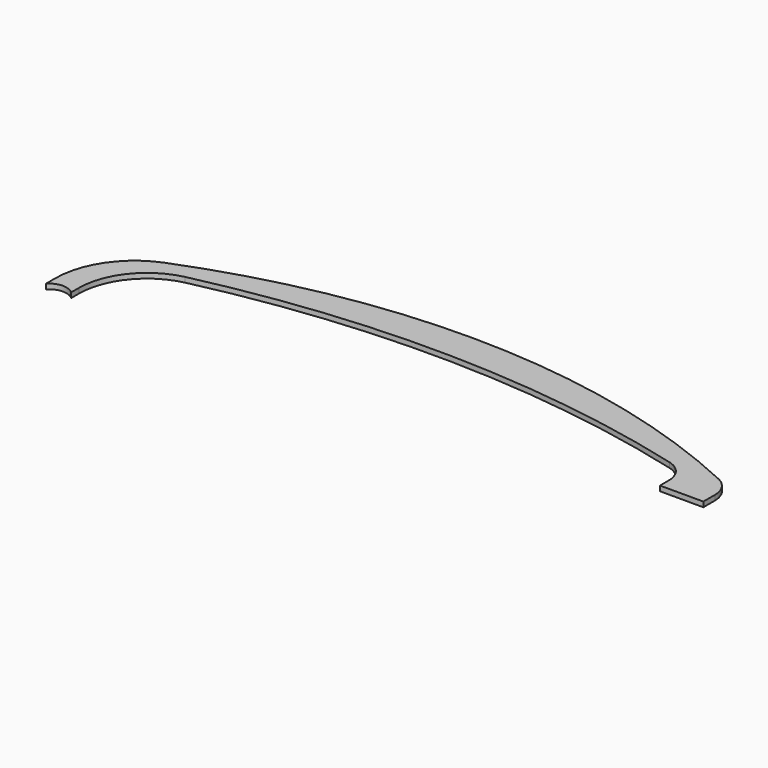
from build123d import *

# Parameters (mm, degrees)
F1_DEPTH = 4
F2_R     = 54.0232948569
F3_R     = 62.809614709
F4_W     = 34.3843554476
F4_H     = 20.342006709
F5_DEPTH = 4
F7_R     = 20


with BuildPart() as f1:
    # F0 (on Top) → F1 (new body)
    with BuildSketch(Plane.XY):
        with BuildLine():
            ThreePointArc((-214.4679278135, 0), (8.6127225609, 31.0011100466), (231.6933729353, 0))
            Line((231.6933729353, 0), (231.6933729353, -24.0185298026))
            Line((231.6933729353, -24.0185298026), (266.0777283828, -24.0185298026))
            Line((266.0777283828, -24.0185298026), (266.0777283828, 0))
            ThreePointArc((266.0777283828, 0), (16.0777283828, 58.0256148842), (-233.9222716172, 0))
            Line((-233.9222716172, 0), (-233.9222716172, -50))
            ThreePointArc((-233.9222716172, -50), (-224.3045684517, -45.7747103429), (-214.4679278135, -49.461685773))
            Line((-214.4679278135, -49.461685773), (-214.4679278135, 0))
        make_face()
    extrude(amount=F1_DEPTH)

    # F2
    f2_edges = [f1.edges().sort_by_distance(p)[0] for p in [
        (-214.467928, 0, 2),
    ]]
    fillet(f2_edges, radius=F2_R)

    # F3
    f3_edges = [f1.edges().sort_by_distance(p)[0] for p in [
        (-233.922272, 0, 2),
    ]]
    fillet(f3_edges, radius=F3_R)

    # F7
    f7_edges = [f1.edges().sort_by_distance(p)[0] for p in [
        (266.077728, 0, 2),
        (231.693373, 0, 2),
    ]]
    fillet(f7_edges, radius=F7_R)


with BuildPart() as f5:
    # F4 (on face) → F5 (new body)
    with BuildSketch(Plane.XY.offset(4)):
        with Locations((248.885550659, -10.1710033545)):
            Rectangle(F4_W, F4_H)
    extrude(amount=F5_DEPTH)


solid = f1.part
